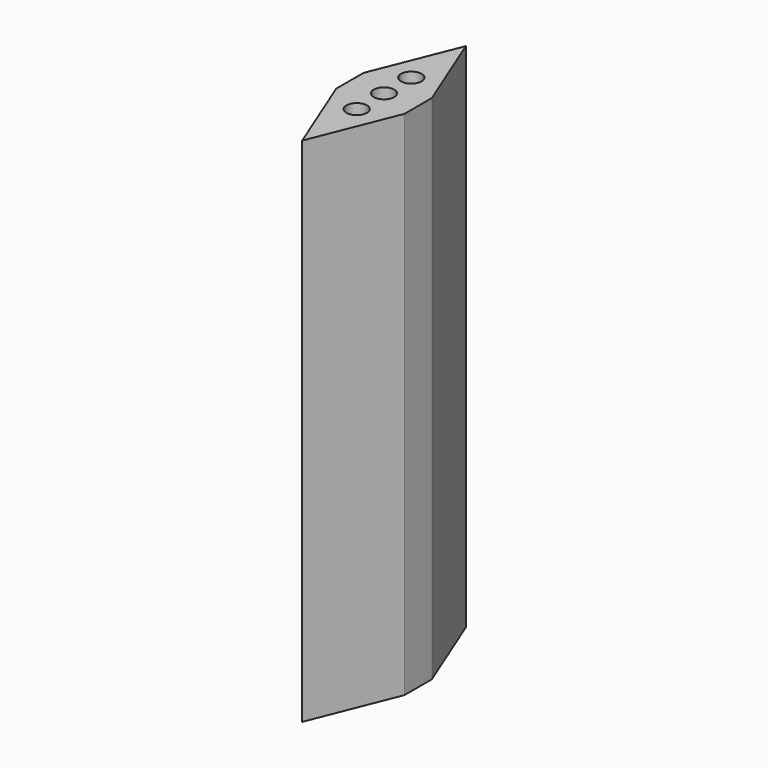
from build123d import *

# Parameters (mm, degrees)
F0_W       = 20
F0_H       = 60
F1_DEPTH   = 150
F2_D       = 6
F2_DEPTH   = 150
F2_TIP     = 1.8025818571
F3_SIZE2   = 10
F3_SIZE    = 25
F3_2_SIZE2 = 9.99999
F3_2_SIZE  = 24.99999


# Not quite as in the source:
# - a fillet or chamfer is up to 0.001 mm smaller than in the source, because OpenCascade refuses the exact size


with BuildPart() as f1:
    # F0 (on Top) → F1 (new body)
    with BuildSketch(Plane.XY):
        Rectangle(F0_W, F0_H)
    extrude(amount=F1_DEPTH)

    # F2
    with Locations(Plane(origin=(0, 0, 0), x_dir=(1, 0, 0), z_dir=(0, 0, -1))):
        with Locations((0, -10), (0, 0), (0, 10)):
            Hole(F2_D / 2, depth=F2_DEPTH)
            with Locations((0, 0, -(F2_DEPTH + F2_TIP / 2))):  # 118° drill point
                Cone(0, F2_D / 2, F2_TIP, mode=Mode.SUBTRACT)

    # F3
    f3_edges = [f1.edges().sort_by_distance(p)[0] for p in [
        (-10, 30, 75),
        (-10, -30, 75),
    ]]
    f3_side = f1.faces().sort_by_distance((-10, 0, 75))[0]
    chamfer(f3_edges, length=F3_SIZE, length2=F3_SIZE2, reference=f3_side)

    # F3#2 (size 25 and 10 in the source; OpenCascade refuses exactly that, so slightly less here)
    f3_2_edges = [f1.edges().sort_by_distance(p)[0] for p in [
        (10, -30, 75),
        (10, 30, 75),
    ]]
    f3_2_side = f1.faces().sort_by_distance((10, 0, 75))[0]
    chamfer(f3_2_edges, length=F3_2_SIZE, length2=F3_2_SIZE2, reference=f3_2_side)


solid = f1.part
